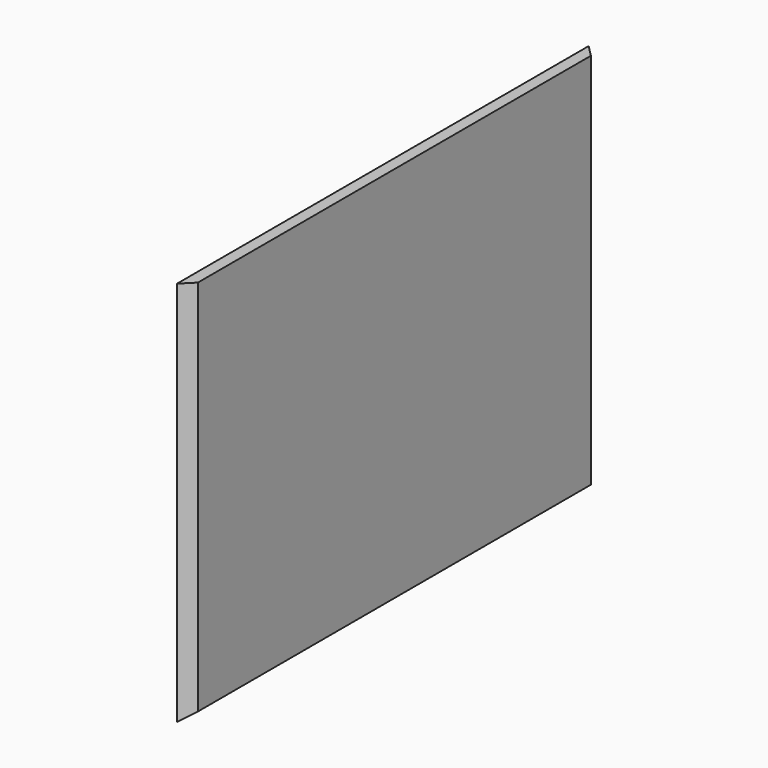
from build123d import *

# Parameters (mm, degrees)
F0_W     = 400
F0_H     = 300
F1_DEPTH = 9
F3_DEPTH = 300
F5_DEPTH = 400
F6_DEPTH = 30


# Not quite as in the source:
# - a feature names something its author has since deleted; it is built from what else it names


with BuildPart() as f1:
    # F0 (on Right) → F1 (new body)
    with BuildSketch(Plane.YZ):
        with Locations((176.1937195063, 136.9389362159)):
            Rectangle(F0_W, F0_H)
    extrude(amount=F1_DEPTH)

    # F2 (on face) → F3 (cut)
    with BuildSketch(Plane.XY.offset(286.9389362159)):
        Polygon((9, 376.1937195063), (0, 376.1937195063), (9, 367.1937195063), align=None)
        Polygon((9, -14.8062804937), (0, -23.8062804937), (9, -23.8062804937), align=None)
    extrude(amount=-F3_DEPTH, mode=Mode.SUBTRACT)

    # F4 (on Front) → F5 (cut)
    with BuildSketch(Plane.XZ):
        Polygon((9, -6.68870858), (0, -13.0610637841), (9, -13.0610637841), align=None)
    extrude(amount=-F5_DEPTH, mode=Mode.SUBTRACT)

    # F4 (on Front) → F6 (cut)
    with BuildSketch(Plane.XZ):
        Polygon((9, -6.68870858), (0, -13.0610637841), (9, -13.0610637841), align=None)
    extrude(amount=F6_DEPTH, mode=Mode.SUBTRACT)


solid = f1.part
